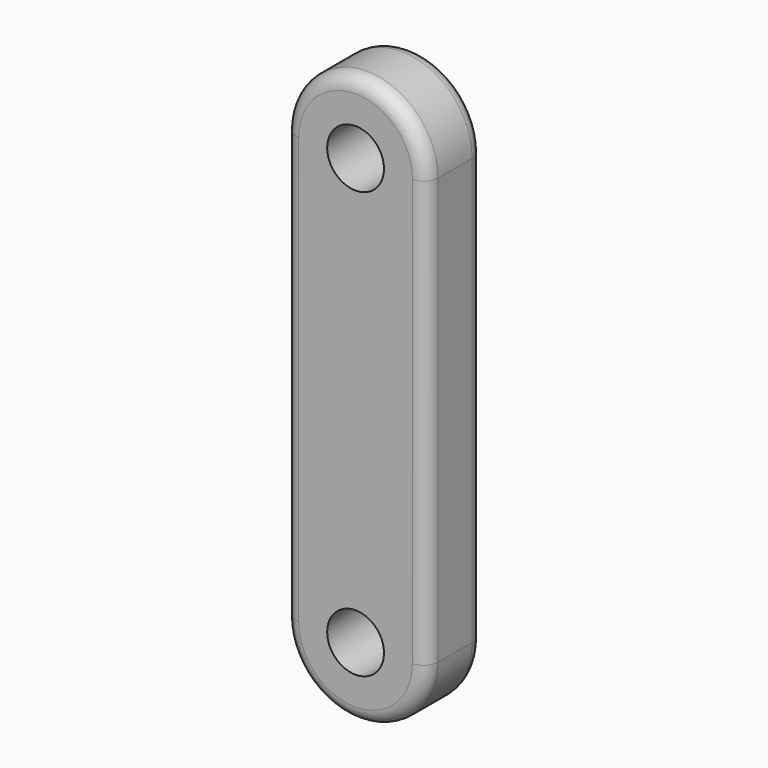
from build123d import *

# Parameters (mm, degrees)
F0_W     = 10
F0_H     = 30
F1_DEPTH = 5
F3_D     = 4
F4_R     = 1


# Not quite as in the source:
# - a feature of the source that left no trace in its solid (it failed there, or was rolled back) is left out


with BuildPart() as f1:
    # F0 (on Front) → F1 (new body)
    with BuildSketch(Plane.XZ):
        with BuildLine():
            Line((5, -15), (-5, -15))
            ThreePointArc((-5, -15), (0, -20), (5, -15))
        make_face()
        with BuildLine():
            ThreePointArc((5, 15), (0, 20), (-5, 15))
            Line((-5, 15), (5, 15))
        make_face()
        Rectangle(F0_W, F0_H)
    extrude(amount=F1_DEPTH)

    # F3 (through all)
    with Locations(Plane(origin=(0, 0, 0), x_dir=(1, 0, 0), z_dir=(0, 1, 0))):
        with Locations((0, -15), (0, 15)):
            Hole(F3_D / 2)

    # F4
    f4_edges = [f1.edges().sort_by_distance(p)[0] for p in [
        (5, -5, 0),
        (5, 0, 0),
        (0, 0, -20),
        (0, -5, -20),
        (-5, 0, 0),
        (-5, -5, 0),
        (0, 0, 20),
        (0, -5, 20),
    ]]
    fillet(f4_edges, radius=F4_R)


solid = f1.part
